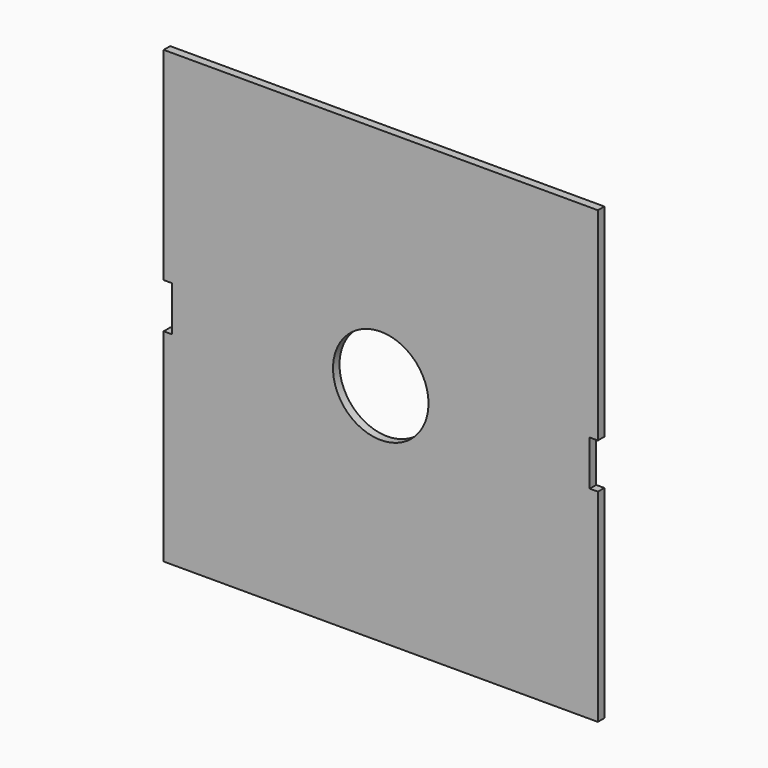
from build123d import *

# Parameters (mm, degrees)
F0_R     = 16.1544
F1_DEPTH = 2.7432


# Not quite as in the source:
# - a feature names something its author has since deleted; it is built from what else it names


with BuildPart() as f1:
    # F0 (on Front) → F1 (new body)
    with BuildSketch(Plane.XZ):
        Polygon((-15.24, 118.095377792), (-81.0768, 118.095377792), (-81.0768, 49.515377792), (-78.3336, 49.515377792), (-78.3336, 34.275377792), (-81.0768, 34.275377792), (-81.0768, -34.304622208), (-15.24, -34.304622208), (0, -34.304622208), (65.8114, -34.304622208), (65.8114, 34.275377792), (63.0682, 34.275377792), (63.0682, 49.515377792), (65.8114, 49.515377792), (65.8114, 118.095377792), (0, 118.095377792), align=None)
        with Locations((-7.6327, 41.895377792)):
            Circle(F0_R, mode=Mode.SUBTRACT)
    extrude(amount=F1_DEPTH)


solid = f1.part
